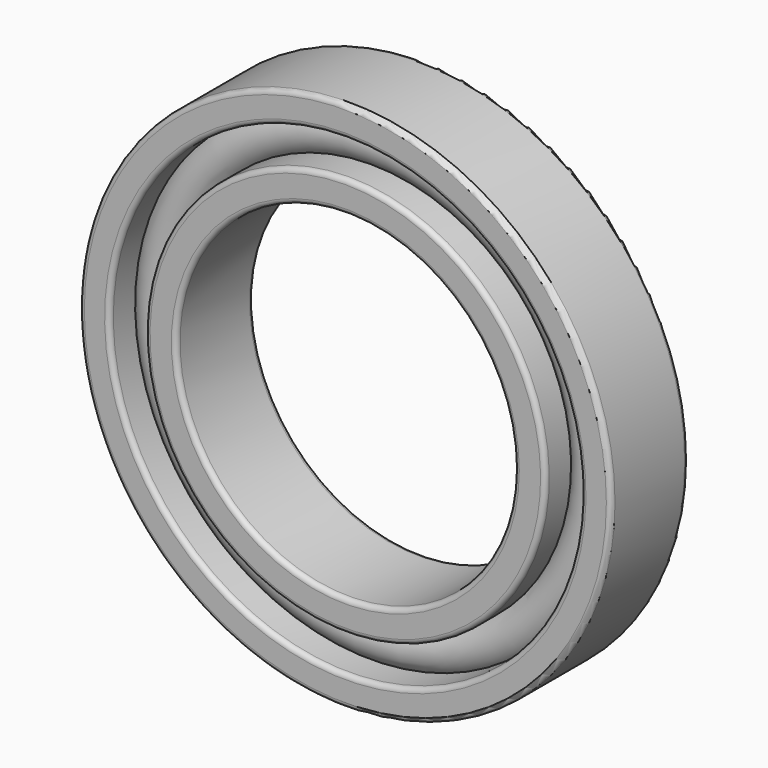
from build123d import *

# Parameters (mm, degrees)
F0_R     = 55
F0_R_2   = 35
F1_DEPTH = 10
F4_R     = 1


with BuildPart() as f1:
    # F0 (on Front) → F1 (new body, symmetric)
    with BuildSketch(Plane.XZ):
        Circle(F0_R)
        Circle(F0_R_2, mode=Mode.SUBTRACT)
    extrude(amount=F1_DEPTH, both=True)

    # F2 (on Right) → F3 (revolve, cut)
    with BuildSketch(Plane.YZ):
        with BuildLine():
            Line((-3.3630343442, 48.8), (-20, 48.8))
            Line((-20, 48.8), (-20, 41.4))
            Line((-20, 41.4), (-3.3630343442, 41.4))
            ThreePointArc((-3.3630343442, 41.4), (-5, 45.1), (-3.3630343442, 48.8))
        make_face()
        with BuildLine():
            Line((20, 41.4), (20, 48.8))
            Line((20, 48.8), (3.3630343442, 48.8))
            ThreePointArc((3.3630343442, 48.8), (5, 45.1), (3.3630343442, 41.4))
            Line((3.3630343442, 41.4), (20, 41.4))
        make_face()
    revolve(axis=Axis((0, 16.4881043163, 0), (0, 1, 0)), mode=Mode.SUBTRACT)

    # F4
    f4_edges = [f1.edges().sort_by_distance(p)[0] for p in [
        (-55, 10, 0),
        (-55, -10, 0),
        (-35, 10, 0),
        (-35, -10, 0),
        (0, -10, -48.8),
        (0, -10, -41.4),
        (0, 10, -48.8),
        (0, 10, -41.4),
    ]]
    fillet(f4_edges, radius=F4_R)


solid = f1.part
